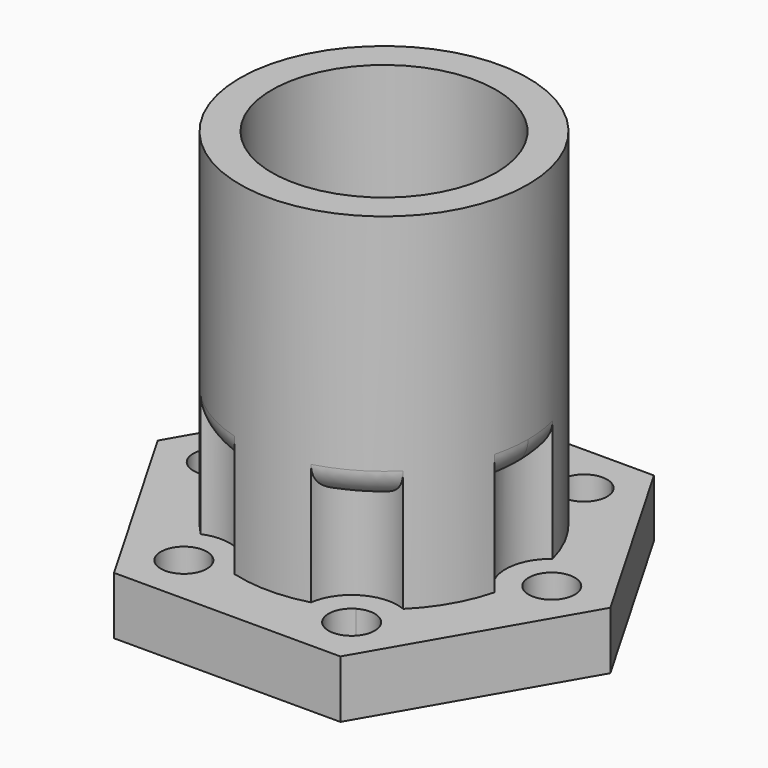
from build123d import *

# Parameters (mm, degrees)
F1_DEPTH      = 5
F2_R          = 12.5
F3_DEPTH      = 30
F4_R          = 9.725
F5_DEPTH      = 29
F6_R          = 6
F7_DEPTH      = 25.4
F9_DEPTH      = 25.4
F10_R         = 4
F11_DEPTH     = 8
F12_T4_ANGLE  = 87.4800969246
F12_S5_R      = 4
F12_T6_DEPTH  = 12
F12_T10_ANGLE = 87.4800969246
F12_S11_R     = 4
F12_T12_DEPTH = 11
F12_T16_ANGLE = 87.4800969246
F12_S17_R     = 4
F12_T18_DEPTH = 11
F12_T22_ANGLE = 43.739121488
F12_S23_R     = 4
F12_T24_DEPTH = 8
F12_T28_ANGLE = 43.739121488
F12_S29_R     = 4
F12_T30_DEPTH = 8
F12_T34_ANGLE = 87.4800969246
F12_S35_R     = 4
F12_T36_DEPTH = 11
F12_T40_ANGLE = 87.4800969246
F12_S41_R     = 4
F12_T42_DEPTH = 11


# Not quite as in the source:
# - a fillet or chamfer that OpenCascade refuses, or shapes differently, is made with other operations: its cross-section is extruded or revolved along the edge and cut away or added


with BuildPart() as f1:
    # F0 (on Top) → F1 (new body)
    with BuildSketch(Plane.XY):
        Polygon((9.8149545762, 17), (-9.8149545762, 17), (-19.6299091524, 0), (-9.8149545762, -17), (9.8149545762, -17), (19.6299091524, 0), align=None)
    extrude(amount=F1_DEPTH)

    # F2 (on face) → F3 (join)
    with BuildSketch(Plane.XY.offset(5)):
        Circle(F2_R)
    extrude(amount=F3_DEPTH)

    # F4 (on face) → F5 (cut)
    with BuildSketch(Plane.XY.offset(35)):
        Circle(F4_R)
    extrude(amount=-F5_DEPTH, mode=Mode.SUBTRACT)

    # F6 (on face) → F7 (cut)
    with BuildSketch(Plane(origin=(0, 0, 0), x_dir=(1, 0, 0), z_dir=(0, 0, -1))):
        Circle(F6_R)
    extrude(amount=-F7_DEPTH, mode=Mode.SUBTRACT)

    # F8 (on face) → F9 (cut)
    with BuildSketch(Plane.XY.offset(5)):
        with BuildLine():
            ThreePointArc((-6.2749545762, 10.8685401412), (-5.5429037687, 11.6005909488), (-5.2749545762, 12.6005909488))
            ThreePointArc((-5.2749545762, 12.6005909488), (-6.2749545762, 14.3326417563), (-8.2749545762, 14.3326417563))
            Line((-8.2749545762, 14.3326417563), (-6.2749545762, 10.8685401412))
        make_face()
        with BuildLine():
            ThreePointArc((8.2749545762, 14.3326417563), (5.5429037687, 13.6005909488), (6.2749545762, 10.8685401412))
            Line((6.2749545762, 10.8685401412), (8.2749545762, 14.3326417563))
        make_face()
        with BuildLine():
            Line((8.2749545762, 14.3326417563), (6.2749545762, 10.8685401412))
            ThreePointArc((6.2749545762, 10.8685401412), (8.2749545762, 10.8685401412), (9.2749545762, 12.6005909488))
            ThreePointArc((9.2749545762, 12.6005909488), (9.0070053838, 13.6005909488), (8.2749545762, 14.3326417563))
        make_face()
        with BuildLine():
            ThreePointArc((16.5499091524, 0), (14.5499091524, 2), (12.5499091524, 0))
            Line((12.5499091524, 0), (16.5499091524, 0))
        make_face()
        with BuildLine():
            Line((16.5499091524, 0), (12.5499091524, 0))
            ThreePointArc((12.5499091524, 0), (14.5499091524, -2), (16.5499091524, 0))
        make_face()
        with BuildLine():
            ThreePointArc((9.2749545762, -12.6005909488), (8.2749545762, -10.8685401412), (6.2749545762, -10.8685401412))
            Line((6.2749545762, -10.8685401412), (8.2749545762, -14.3326417563))
            ThreePointArc((8.2749545762, -14.3326417563), (9.0070053838, -13.6005909488), (9.2749545762, -12.6005909488))
        make_face()
        with BuildLine():
            Line((8.2749545762, -14.3326417563), (6.2749545762, -10.8685401412))
            ThreePointArc((6.2749545762, -10.8685401412), (5.5429037687, -13.6005909488), (8.2749545762, -14.3326417563))
        make_face()
        with BuildLine():
            ThreePointArc((-5.2749545762, -12.6005909488), (-5.5429037687, -11.6005909488), (-6.2749545762, -10.8685401412))
            Line((-6.2749545762, -10.8685401412), (-8.2749545762, -14.3326417563))
            ThreePointArc((-8.2749545762, -14.3326417563), (-6.2749545762, -14.3326417563), (-5.2749545762, -12.6005909488))
        make_face()
        with BuildLine():
            Line((-8.2749545762, -14.3326417563), (-6.2749545762, -10.8685401412))
            ThreePointArc((-6.2749545762, -10.8685401412), (-9.0070053838, -11.6005909488), (-8.2749545762, -14.3326417563))
        make_face()
        with BuildLine():
            ThreePointArc((-16.5499091524, 0), (-14.5499091524, -2), (-12.5499091524, 0))
            Line((-12.5499091524, 0), (-16.5499091524, 0))
        make_face()
        with BuildLine():
            Line((-16.5499091524, 0), (-12.5499091524, 0))
            ThreePointArc((-12.5499091524, 0), (-14.5499091524, 2), (-16.5499091524, 0))
        make_face()
        with BuildLine():
            Line((-6.2749545762, 10.8685401412), (-8.2749545762, 14.3326417563))
            ThreePointArc((-8.2749545762, 14.3326417563), (-9.0070053838, 11.6005909488), (-6.2749545762, 10.8685401412))
        make_face()
    extrude(amount=-F9_DEPTH, mode=Mode.SUBTRACT)

    # F10 (on face) → F11 (cut)
    with BuildSketch(Plane.XY.offset(5)):
        with Locations((-7.2749545762, -12.6005909488)):
            Circle(F10_R)
        with Locations((-14.5499091524, 0)):
            Circle(F10_R)
        with Locations((-7.2749545762, 12.6005909488)):
            Circle(F10_R)
        with Locations((7.2749545762, 12.6005909488)):
            Circle(F10_R)
        with Locations((14.5499091524, 0)):
            Circle(F10_R)
        with Locations((7.2749545762, -12.6005909488)):
            Circle(F10_R)
    extrude(amount=F11_DEPTH, mode=Mode.SUBTRACT)

    # F12: fillet of radius 2.54 on 7 edges, made by hand


with BuildPart() as f12_tool2:
    # F12_s3 → F12_t4 (revolve)
    with BuildSketch(Plane(origin=(0, 0, 0), x_dir=(0, 0, 1), z_dir=(0.6913875801, -0.7224840581, 0))):
        with BuildLine():
            ThreePointArc((13, 9.96), (13.7439487758, 11.7560512242), (15.54, 12.5))
            Line((15.54, 12.5), (13, 12.5))
            Line((13, 12.5), (13, 9.96))
        make_face()
    revolve(axis=Axis((0, 0, 13), (0, 0, -1)), revolution_arc=F12_T4_ANGLE)

    # F12_s5 → F12_t6 (intersect, symmetric)
    with BuildSketch(Plane.XY.offset(15.2)):
        with Locations((-14.5499091524, 0)):
            Circle(F12_S5_R)
    extrude(amount=F12_T6_DEPTH, both=True, mode=Mode.INTERSECT)


with BuildPart() as f1_1:
    add(f1.part)

    # F12_t1: cut F12_tool2
    add(f12_tool2.part, mode=Mode.SUBTRACT)


with BuildPart() as f12_tool8:
    # F12_s9 → F12_t10 (revolve)
    with BuildSketch(Plane(origin=(0, 0, 0), x_dir=(0, 0, 1), z_dir=(0.9713833381, 0.2375171792, 0))):
        with BuildLine():
            ThreePointArc((13, 9.96), (13.7439487758, 11.7560512242), (15.54, 12.5))
            Line((15.54, 12.5), (13, 12.5))
            Line((13, 12.5), (13, 9.96))
        make_face()
    revolve(axis=Axis((0, 0, 13), (0, 0, -1)), revolution_arc=F12_T10_ANGLE)

    # F12_s11 → F12_t12 (intersect, symmetric)
    with BuildSketch(Plane.XY.offset(15.2)):
        with Locations((-7.2749545762, -12.6005909488)):
            Circle(F12_S11_R)
    extrude(amount=F12_T12_DEPTH, both=True, mode=Mode.INTERSECT)


with BuildPart() as f1_2:
    add(f1_1.part)

    # F12_t7: cut F12_tool8
    add(f12_tool8.part, mode=Mode.SUBTRACT)


with BuildPart() as f12_tool14:
    # F12_s15 → F12_t16 (revolve)
    with BuildSketch(Plane(origin=(0, 0, 0), x_dir=(0, 0, 1), z_dir=(0.2799957581, 0.9600012372, 0))):
        with BuildLine():
            ThreePointArc((13, 9.96), (13.7439487758, 11.7560512242), (15.54, 12.5))
            Line((15.54, 12.5), (13, 12.5))
            Line((13, 12.5), (13, 9.96))
        make_face()
    revolve(axis=Axis((0, 0, 13), (0, 0, -1)), revolution_arc=F12_T16_ANGLE)

    # F12_s17 → F12_t18 (intersect, symmetric)
    with BuildSketch(Plane.XY.offset(15.2)):
        with Locations((7.2749545762, -12.6005909488)):
            Circle(F12_S17_R)
    extrude(amount=F12_T18_DEPTH, both=True, mode=Mode.INTERSECT)


with BuildPart() as f1_3:
    add(f1_2.part)

    # F12_t13: cut F12_tool14
    add(f12_tool14.part, mode=Mode.SUBTRACT)


with BuildPart() as f12_tool20:
    # F12_s21 → F12_t22 (revolve)
    with BuildSketch(Plane(origin=(0, 0, 0), x_dir=(0, 0, 1), z_dir=(-0.6913758911, 0.7224952438, 0))):
        with BuildLine():
            ThreePointArc((13, 9.96), (13.7439487758, 11.7560512242), (15.54, 12.5))
            Line((15.54, 12.5), (13, 12.5))
            Line((13, 12.5), (13, 9.96))
        make_face()
    revolve(axis=Axis((0, 0, 13), (0, 0, -1)), revolution_arc=F12_T22_ANGLE)

    # F12_s23 → F12_t24 (intersect, symmetric)
    with BuildSketch(Plane.XY.offset(15.2)):
        with Locations((14.5499091524, 0)):
            Circle(F12_S23_R)
    extrude(amount=F12_T24_DEPTH, both=True, mode=Mode.INTERSECT)


with BuildPart() as f1_4:
    add(f1_3.part)

    # F12_t19: cut F12_tool20
    add(f12_tool20.part, mode=Mode.SUBTRACT)


with BuildPart() as f12_tool26:
    # F12_s27 → F12_t28 (revolve)
    with BuildSketch(Plane.XZ):
        with BuildLine():
            ThreePointArc((9.96, 13), (11.7560512242, 13.7439487758), (12.5, 15.54))
            Line((12.5, 15.54), (12.5, 13))
            Line((12.5, 13), (9.96, 13))
        make_face()
    revolve(axis=Axis((0, 0, 13), (0, 0, -1)), revolution_arc=F12_T28_ANGLE)

    # F12_s29 → F12_t30 (intersect, symmetric)
    with BuildSketch(Plane.XY.offset(15.2)):
        with Locations((14.5499091524, 0)):
            Circle(F12_S29_R)
    extrude(amount=F12_T30_DEPTH, both=True, mode=Mode.INTERSECT)


with BuildPart() as f1_5:
    add(f1_4.part)

    # F12_t25: cut F12_tool26
    add(f12_tool26.part, mode=Mode.SUBTRACT)


with BuildPart() as f12_tool32:
    # F12_s33 → F12_t34 (revolve)
    with BuildSketch(Plane(origin=(0, 0, 0), x_dir=(0, 0, 1), z_dir=(-0.9713833381, -0.2375171792, 0))):
        with BuildLine():
            ThreePointArc((13, 9.96), (13.7439487758, 11.7560512242), (15.54, 12.5))
            Line((15.54, 12.5), (13, 12.5))
            Line((13, 12.5), (13, 9.96))
        make_face()
    revolve(axis=Axis((0, 0, 13), (0, 0, -1)), revolution_arc=F12_T34_ANGLE)

    # F12_s35 → F12_t36 (intersect, symmetric)
    with BuildSketch(Plane.XY.offset(15.2)):
        with Locations((7.2749545762, 12.6005909488)):
            Circle(F12_S35_R)
    extrude(amount=F12_T36_DEPTH, both=True, mode=Mode.INTERSECT)


with BuildPart() as f1_6:
    add(f1_5.part)

    # F12_t31: cut F12_tool32
    add(f12_tool32.part, mode=Mode.SUBTRACT)


with BuildPart() as f12_tool38:
    # F12_s39 → F12_t40 (revolve)
    with BuildSketch(Plane(origin=(0, 0, 0), x_dir=(0, 0, 1), z_dir=(-0.2799957581, -0.9600012372, 0))):
        with BuildLine():
            ThreePointArc((13, 9.96), (13.7439487758, 11.7560512242), (15.54, 12.5))
            Line((15.54, 12.5), (13, 12.5))
            Line((13, 12.5), (13, 9.96))
        make_face()
    revolve(axis=Axis((0, 0, 13), (0, 0, -1)), revolution_arc=F12_T40_ANGLE)

    # F12_s41 → F12_t42 (intersect, symmetric)
    with BuildSketch(Plane.XY.offset(15.2)):
        with Locations((-7.2749545762, 12.6005909488)):
            Circle(F12_S41_R)
    extrude(amount=F12_T42_DEPTH, both=True, mode=Mode.INTERSECT)


with BuildPart() as f1_7:
    add(f1_6.part)

    # F12_t37: cut F12_tool38
    add(f12_tool38.part, mode=Mode.SUBTRACT)


solid = f1_7.part
